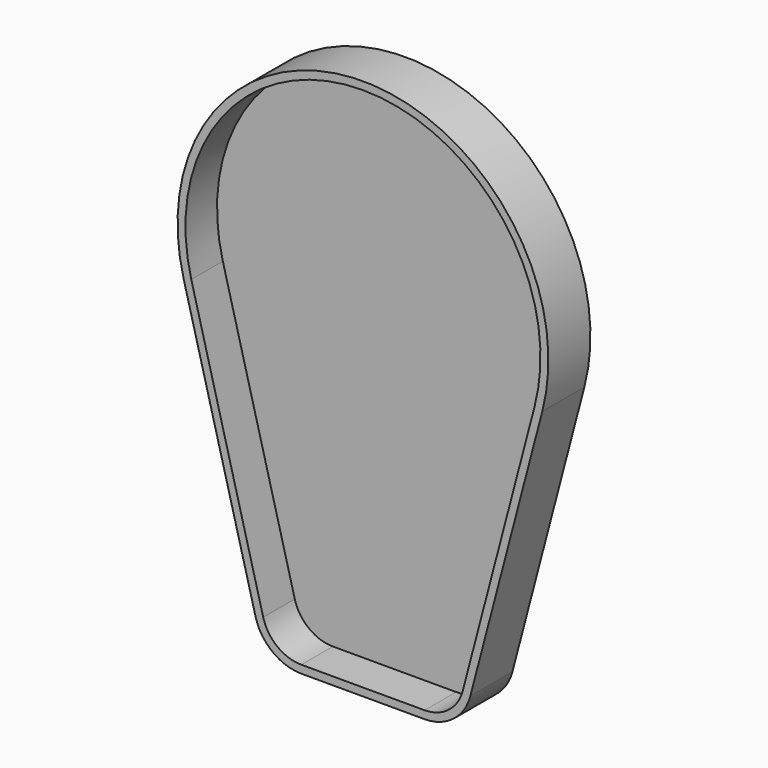
from build123d import *

# Parameters (mm, degrees)
F1_DEPTH = 508
F2_DEPTH = 381


# Not quite as in the source:
# - a feature of the source that left no trace in its solid (it failed there, or was rolled back) is left out


with BuildPart() as f1:
    # F0 (on Front) → F1 (new body)
    with BuildSketch(Plane.XZ):
        with BuildLine():
            Line((1456.3986319797, -1504.4493615516), (1731.9998491091, -454.7340021221))
            ThreePointArc((1731.9998491091, -454.7340021221), (0, 1790.7), (-1731.9998491091, -454.7340021221))
            Line((-1731.9998491091, -454.7340021221), (-1456.3986319797, -1504.4493615516))
            Line((-1456.3986319797, -1504.4493615516), (-1356.3676447382, -1885.4493615516))
            Line((-1356.3676447382, -1885.4493615516), (-1156.3056702552, -2647.4493615516))
            Line((-1156.3056702552, -2647.4493615516), (-1056.2746830137, -3028.4493615516))
            Line((-1056.2746830137, -3028.4493615516), (-1037.3310360144, -3100.6022984142))
            ThreePointArc((-1037.3310360144, -3100.6022984142), (-874.3582315562, -3346.5178247234), (-595.1183085823, -3441.7))
            Line((-595.1183085823, -3441.7), (595.1183085823, -3441.7))
            ThreePointArc((595.1183085823, -3441.7), (874.3582315562, -3346.5178247234), (1037.3310360144, -3100.6022984142))
            Line((1037.3310360144, -3100.6022984142), (1056.2746830137, -3028.4493615516))
            Line((1056.2746830137, -3028.4493615516), (1156.3056702552, -2647.4493615516))
            Line((1156.3056702552, -2647.4493615516), (1356.3676447382, -1885.4493615516))
            Line((1356.3676447382, -1885.4493615516), (1456.3986319797, -1504.4493615516))
        make_face()
        with BuildLine():
            ThreePointArc((-1658.2977278704, -435.3836190531), (0, 1714.5), (1658.2977278704, -435.3836190531))
            Line((1658.2977278704, -435.3836190531), (963.6289147757, -3081.2519153451))
            ThreePointArc((963.6289147757, -3081.2519153451), (827.8182443939, -3286.1815206028), (595.1183085823, -3365.5))
            Line((595.1183085823, -3365.5), (-595.1183085823, -3365.5))
            ThreePointArc((-595.1183085823, -3365.5), (-827.8182443939, -3286.1815206028), (-963.6289147757, -3081.2519153451))
            Line((-963.6289147757, -3081.2519153451), (-1658.2977278704, -435.3836190531))
        make_face(mode=Mode.SUBTRACT)
        with BuildLine():
            Line((963.6289147757, -3081.2519153451), (1658.2977278704, -435.3836190531))
            ThreePointArc((1658.2977278704, -435.3836190531), (0, 1714.5), (-1658.2977278704, -435.3836190531))
            Line((-1658.2977278704, -435.3836190531), (-963.6289147757, -3081.2519153451))
            ThreePointArc((-963.6289147757, -3081.2519153451), (-827.8182443939, -3286.1815206028), (-595.1183085823, -3365.5))
            Line((-595.1183085823, -3365.5), (595.1183085823, -3365.5))
            ThreePointArc((595.1183085823, -3365.5), (827.8182443939, -3286.1815206028), (963.6289147757, -3081.2519153451))
        make_face()
    extrude(amount=-F1_DEPTH)

    # F0 (on Front) → F2 (cut)
    with BuildSketch(Plane.XZ):
        with BuildLine():
            Line((963.6289147757, -3081.2519153451), (1658.2977278704, -435.3836190531))
            ThreePointArc((1658.2977278704, -435.3836190531), (0, 1714.5), (-1658.2977278704, -435.3836190531))
            Line((-1658.2977278704, -435.3836190531), (-963.6289147757, -3081.2519153451))
            ThreePointArc((-963.6289147757, -3081.2519153451), (-827.8182443939, -3286.1815206028), (-595.1183085823, -3365.5))
            Line((-595.1183085823, -3365.5), (595.1183085823, -3365.5))
            ThreePointArc((595.1183085823, -3365.5), (827.8182443939, -3286.1815206028), (963.6289147757, -3081.2519153451))
        make_face()
    extrude(amount=-F2_DEPTH, mode=Mode.SUBTRACT)


solid = f1.part
